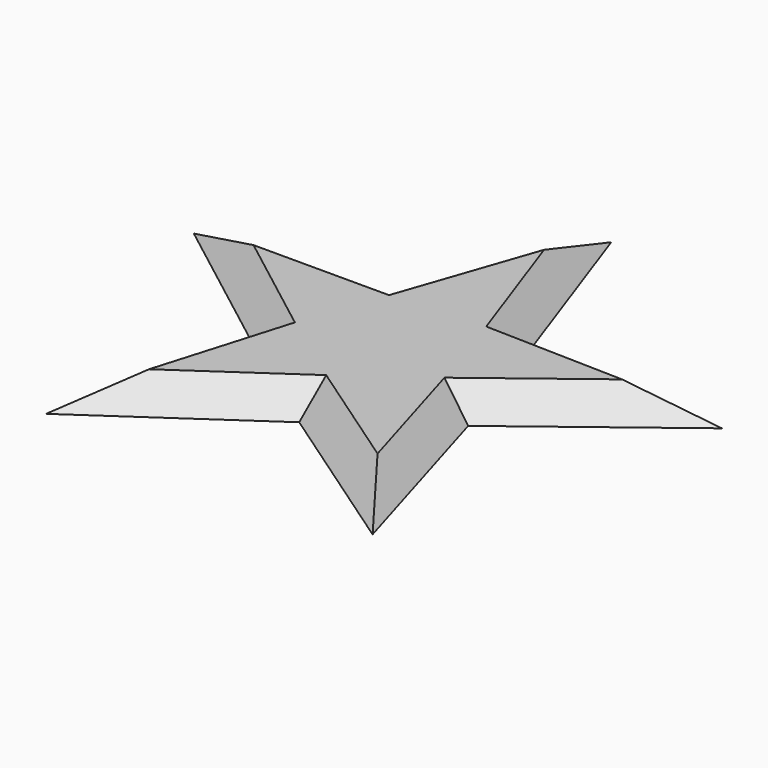
from build123d import *

# Parameters (mm, degrees)
F1_DEPTH      = 5
F2_T4_DEPTH   = 68.6680055615
F2_T9_DEPTH   = 69.5804590238
F2_T14_DEPTH  = 68.6556539851
F2_T19_DEPTH  = 68.6680055615
F2_T24_DEPTH  = 68.6680055615
F2_T29_DEPTH  = 68.6680055615
F2_T34_DEPTH  = 68.6680055615
F2_T39_DEPTH  = 68.6680055615
F2_T44_DEPTH  = 68.6680055615
F2_T49_DEPTH  = 68.6680055615
F2_T55_DEPTH  = 68.6680055615
F2_T59_DEPTH  = 68.6680055615
F2_T66_DEPTH  = 69.5804590238
F2_T70_DEPTH  = 68.6556539851
F2_T77_DEPTH  = 68.6680055615
F2_T81_DEPTH  = 68.6680055615
F2_T88_DEPTH  = 68.6680055615
F2_T92_DEPTH  = 68.6680055615
F2_T99_DEPTH  = 68.6680055615
F2_T103_DEPTH = 68.6680055615


# Not quite as in the source:
# - a fillet or chamfer that OpenCascade refuses, or shapes differently, is made with other operations: its cross-section is extruded or revolved along the edge and cut away or added


with BuildPart() as f1:
    # F0 (on Top) → F1 (new body)
    with BuildSketch(Plane.XY):
        Polygon((0, 0), (0, 52.987328628), (-12.5984860432, 16.3739850326), align=None)
        Polygon((12.5984860432, 17.3403284151), (0, 52.987328628), (0, 0), align=None)
        Polygon((0, 0), (-12.5984860432, 16.3739850326), (-50.3939441727, 16.3739850326), align=None)
        Polygon((50.3939441727, 16.3739850326), (12.5984860432, 17.3403284151), (0, 0), align=None)
        Polygon((20.3847786247, -6.6234160785), (0, 0), (31.1451703259, -42.8676493466), align=None)
        Polygon((0, -21.4338246733), (0, 0), (-31.1451703259, -42.8676493466), align=None)
        Polygon((-20.3847786247, -6.6234160785), (0, 0), (-50.3939441727, 16.3739850326), align=None)
        Polygon((50.3939441727, 16.3739850326), (0, 0), (20.3847786247, -6.6234160785), align=None)
        Polygon((31.1451703259, -42.8676493466), (0, 0), (0, -21.4338246733), align=None)
        Polygon((-31.1451703259, -42.8676493466), (0, 0), (-20.3847786247, -6.6234160785), align=None)
    extrude(amount=F1_DEPTH)

    # F2: chamfer of 6 on 10 edges, made by hand


with BuildPart() as f2_tool2:
    # F2_s3 → F2_t4 (new body)
    with BuildSketch(Plane(origin=(1.0926214012, -3.0915361725, 0), x_dir=(0, 0, 1), z_dir=(-0.3332244354, 0.9428475357, 0))):
        Polygon((-1, 17.6566726657), (5, 11.6566726657), (5, 17.6566726657), align=None)
    extrude(amount=F2_T4_DEPTH)

    split(bisect_by=Plane(origin=(0.451293236, 17.6509043406, 0), x_dir=(0, 0, 1), z_dir=(0.025559359, 0.9996733062, 0)), keep=Keep.TOP)


with BuildPart() as f1_1:
    add(f1.part)

    # F2_t1: cut F2_tool2
    add(f2_tool2.part, mode=Mode.SUBTRACT)


with BuildPart() as f2_tool7:
    # F2_s8 → F2_t9 (new body)
    with BuildSketch(Plane(origin=(21.3229816345, 61.9682119253, 0), x_dir=(0, 0, 1), z_dir=(-0.3253719116, -0.9455861247, 0))):
        Polygon((-1, 17.2405884042), (5, 11.2405884042), (5, 17.2405884042), align=None)
    extrude(amount=F2_T9_DEPTH)

    split(bisect_by=Plane.XZ.offset(-16.3739850326), keep=Keep.BOTTOM)


with BuildPart() as f1_2:
    add(f1_1.part)

    # F2_t6: cut F2_tool7
    add(f2_tool7.part, mode=Mode.SUBTRACT)


with BuildPart() as f2_tool12:
    # F2_s13 → F2_t14 (new body)
    with BuildSketch(Plane.YZ.offset(2.8316118846)):
        Polygon((16.3739850326, -1), (10.3739850326, 5), (16.3739850326, 5), align=None)
    extrude(amount=-F2_T14_DEPTH)

    split(bisect_by=Plane(origin=(-16.3024611761, 5.6096032055, 0), x_dir=(0, 0, 1), z_dir=(-0.9455861247, 0.3253719116, 0)), keep=Keep.TOP)


with BuildPart() as f1_3:
    add(f1_2.part)

    # F2_t11: cut F2_tool12
    add(f2_tool12.part, mode=Mode.SUBTRACT)


with BuildPart() as f2_tool17:
    # F2_s18 → F2_t19 (new body)
    with BuildSketch(Plane(origin=(-51.9012195214, 39.7742870116, 0), x_dir=(0, 0, 1), z_dir=(0.7937292793, -0.6082711823, 0))):
        Polygon((-1, 17.6566726657), (5, 11.6566726657), (5, 17.6566726657), align=None)
    extrude(amount=F2_T19_DEPTH)

    split(bisect_by=Plane(origin=(-16.926464871, 5.0252240345, 0), x_dir=(0, 0, 1), z_dir=(-0.9586440884, 0.2846076455, 0)), keep=Keep.TOP)


with BuildPart() as f1_4:
    add(f1_3.part)

    # F2_t16: cut F2_tool17
    add(f2_tool17.part, mode=Mode.SUBTRACT)


with BuildPart() as f2_tool22:
    # F2_s23 → F2_t24 (new body)
    with BuildSketch(Plane(origin=(0.9332100871, 3.1433320482, 0), x_dir=(0, 0, 1), z_dir=(-0.2846076455, -0.9586440884, 0))):
        Polygon((-1, 17.6566726657), (5, 11.6566726657), (5, 17.6566726657), align=None)
    extrude(amount=F2_T24_DEPTH)

    split(bisect_by=Plane(origin=(-10.7400451584, -14.014618069, 0), x_dir=(0, 0, 1), z_dir=(-0.6082711823, -0.7937292793, 0)), keep=Keep.TOP)


with BuildPart() as f1_5:
    add(f1_4.part)

    # F2_t21: cut F2_tool22
    add(f2_tool22.part, mode=Mode.SUBTRACT)


with BuildPart() as f2_tool27:
    # F2_s28 → F2_t29 (new body)
    with BuildSketch(Plane(origin=(-53.8659537043, -37.0700624038, 0), x_dir=(0, 0, 1), z_dir=(0.8237761079, 0.5669152707, 0))):
        Polygon((-1, 17.6566726657), (5, 11.6566726657), (5, 17.6566726657), align=None)
    extrude(amount=F2_T29_DEPTH)

    split(bisect_by=Plane(origin=(-10.0098373636, -14.5451450862, 0), x_dir=(0, 0, 1), z_dir=(-0.5669152707, -0.8237761079, 0)), keep=Keep.TOP)


with BuildPart() as f1_6:
    add(f1_5.part)

    # F2_t26: cut F2_tool27
    add(f2_tool27.part, mode=Mode.SUBTRACT)


with BuildPart() as f2_tool32:
    # F2_s33 → F2_t34 (new body)
    with BuildSketch(Plane(origin=(-2.7011086511, 1.8588785563, 0), x_dir=(0, 0, 1), z_dir=(0.8237761079, -0.5669152707, 0))):
        Polygon((-1, 17.6566726657), (5, 11.6566726657), (5, 17.6566726657), align=None)
    extrude(amount=F2_T34_DEPTH)

    split(bisect_by=Plane(origin=(10.0098373636, -14.5451450862, 0), x_dir=(0, 0, 1), z_dir=(0.5669152707, -0.8237761079, 0)), keep=Keep.TOP)


with BuildPart() as f1_7:
    add(f1_6.part)

    # F2_t31: cut F2_tool32
    add(f2_tool32.part, mode=Mode.SUBTRACT)


with BuildPart() as f2_tool37:
    # F2_s38 → F2_t39 (new body)
    with BuildSketch(Plane(origin=(18.6102292957, -62.6848455422, 0), x_dir=(0, 0, 1), z_dir=(-0.2846076455, 0.9586440884, 0))):
        Polygon((-1, 17.6566726657), (5, 11.6566726657), (5, 17.6566726657), align=None)
    extrude(amount=F2_T39_DEPTH)

    split(bisect_by=Plane(origin=(10.7400451584, -14.014618069, 0), x_dir=(0, 0, 1), z_dir=(0.6082711823, -0.7937292793, 0)), keep=Keep.TOP)


with BuildPart() as f1_8:
    add(f1_7.part)

    # F2_t36: cut F2_tool37
    add(f2_tool37.part, mode=Mode.SUBTRACT)


with BuildPart() as f2_tool42:
    # F2_s43 → F2_t44 (new body)
    with BuildSketch(Plane(origin=(-2.6025870408, -1.9944819195, 0), x_dir=(0, 0, 1), z_dir=(0.7937292793, 0.6082711823, 0))):
        Polygon((-1, 17.6566726657), (5, 11.6566726657), (5, 17.6566726657), align=None)
    extrude(amount=F2_T44_DEPTH)

    split(bisect_by=Plane(origin=(16.926464871, 5.0252240345, 0), x_dir=(0, 0, 1), z_dir=(0.9586440884, 0.2846076455, 0)), keep=Keep.TOP)


with BuildPart() as f1_9:
    add(f1_8.part)

    # F2_t41: cut F2_tool42
    add(f2_tool42.part, mode=Mode.SUBTRACT)


with BuildPart() as f2_tool47:
    # F2_s48 → F2_t49 (new body)
    with BuildSketch(Plane(origin=(65.3677079475, -1.6713027209, 0), x_dir=(0, 0, 1), z_dir=(-0.9996733062, 0.025559359, 0))):
        Polygon((-1, 17.6566726657), (5, 11.6566726657), (5, 17.6566726657), align=None)
    extrude(amount=F2_T49_DEPTH)

    split(bisect_by=Plane(origin=(16.6475503122, 5.8836347802, 0), x_dir=(0, 0, 1), z_dir=(0.9428475357, 0.3332244354, 0)), keep=Keep.TOP)


with BuildPart() as f1_10:
    add(f1_9.part)

    # F2_t46: cut F2_tool47
    add(f2_tool47.part, mode=Mode.SUBTRACT)


with BuildPart() as f2_tool53:
    # F2_s54 → F2_t55 (new body)
    with BuildSketch(Plane(origin=(1.0926214012, -3.0915361725, 0), x_dir=(0, 0, 1), z_dir=(-0.3332244354, 0.9428475357, 0))):
        Polygon((-1, 17.6566726657), (5, 11.6566726657), (5, 17.6566726657), align=None)
    extrude(amount=F2_T55_DEPTH)

    split(bisect_by=Plane(origin=(0.451293236, 17.6509043406, 0), x_dir=(0, 0, 1), z_dir=(-0.025559359, -0.9996733062, 0)), keep=Keep.TOP)


with BuildPart() as f2_tool57:
    # F2_s58 → F2_t59 (new body)
    with BuildSketch(Plane(origin=(65.3677079475, -1.6713027209, 0), x_dir=(0, 0, 1), z_dir=(-0.9996733062, 0.025559359, 0))):
        Polygon((-1, 17.6566726657), (5, 11.6566726657), (5, 17.6566726657), align=None)
    extrude(amount=F2_T59_DEPTH)

    split(bisect_by=Plane(origin=(16.6475503122, 5.8836347802, 0), x_dir=(0, 0, 1), z_dir=(-0.9428475357, -0.3332244354, 0)), keep=Keep.TOP)


with BuildPart() as f2_tool53_1:
    add(f2_tool53.part)

    # F2_t61: intersect F2_tool57
    add(f2_tool57.part, mode=Mode.INTERSECT)


with BuildPart() as f1_11:
    add(f1_10.part)

    # F2_t51: cut F2_tool53
    add(f2_tool53_1.part, mode=Mode.SUBTRACT)


with BuildPart() as f2_tool64:
    # F2_s65 → F2_t66 (new body)
    with BuildSketch(Plane(origin=(21.3229816345, 61.9682119253, 0), x_dir=(0, 0, 1), z_dir=(-0.3253719116, -0.9455861247, 0))):
        Polygon((-1, 17.2405884042), (5, 11.2405884042), (5, 17.2405884042), align=None)
    extrude(amount=F2_T66_DEPTH)

    split(bisect_by=Plane.XZ.offset(-16.3739850326), keep=Keep.TOP)


with BuildPart() as f2_tool68:
    # F2_s69 → F2_t70 (new body)
    with BuildSketch(Plane.YZ.offset(2.8316118846)):
        Polygon((16.3739850326, -1), (10.3739850326, 5), (16.3739850326, 5), align=None)
    extrude(amount=-F2_T70_DEPTH)

    split(bisect_by=Plane(origin=(-16.3024611761, 5.6096032055, 0), x_dir=(0, 0, 1), z_dir=(0.9455861247, -0.3253719116, 0)), keep=Keep.TOP)


with BuildPart() as f2_tool64_1:
    add(f2_tool64.part)

    # F2_t72: intersect F2_tool68
    add(f2_tool68.part, mode=Mode.INTERSECT)


with BuildPart() as f1_12:
    add(f1_11.part)

    # F2_t62: cut F2_tool64
    add(f2_tool64_1.part, mode=Mode.SUBTRACT)


with BuildPart() as f2_tool75:
    # F2_s76 → F2_t77 (new body)
    with BuildSketch(Plane(origin=(-51.9012195214, 39.7742870116, 0), x_dir=(0, 0, 1), z_dir=(0.7937292793, -0.6082711823, 0))):
        Polygon((-1, 17.6566726657), (5, 11.6566726657), (5, 17.6566726657), align=None)
    extrude(amount=F2_T77_DEPTH)

    split(bisect_by=Plane(origin=(-16.926464871, 5.0252240345, 0), x_dir=(0, 0, 1), z_dir=(0.9586440884, -0.2846076455, 0)), keep=Keep.TOP)


with BuildPart() as f2_tool79:
    # F2_s80 → F2_t81 (new body)
    with BuildSketch(Plane(origin=(0.9332100871, 3.1433320482, 0), x_dir=(0, 0, 1), z_dir=(-0.2846076455, -0.9586440884, 0))):
        Polygon((-1, 17.6566726657), (5, 11.6566726657), (5, 17.6566726657), align=None)
    extrude(amount=F2_T81_DEPTH)

    split(bisect_by=Plane(origin=(-10.7400451584, -14.014618069, 0), x_dir=(0, 0, 1), z_dir=(0.6082711823, 0.7937292793, 0)), keep=Keep.TOP)


with BuildPart() as f2_tool75_1:
    add(f2_tool75.part)

    # F2_t83: intersect F2_tool79
    add(f2_tool79.part, mode=Mode.INTERSECT)


with BuildPart() as f1_13:
    add(f1_12.part)

    # F2_t73: cut F2_tool75
    add(f2_tool75_1.part, mode=Mode.SUBTRACT)


with BuildPart() as f2_tool86:
    # F2_s87 → F2_t88 (new body)
    with BuildSketch(Plane(origin=(-53.8659537043, -37.0700624038, 0), x_dir=(0, 0, 1), z_dir=(0.8237761079, 0.5669152707, 0))):
        Polygon((-1, 17.6566726657), (5, 11.6566726657), (5, 17.6566726657), align=None)
    extrude(amount=F2_T88_DEPTH)

    split(bisect_by=Plane(origin=(-10.0098373636, -14.5451450862, 0), x_dir=(0, 0, 1), z_dir=(0.5669152707, 0.8237761079, 0)), keep=Keep.TOP)


with BuildPart() as f2_tool90:
    # F2_s91 → F2_t92 (new body)
    with BuildSketch(Plane(origin=(-2.7011086511, 1.8588785563, 0), x_dir=(0, 0, 1), z_dir=(0.8237761079, -0.5669152707, 0))):
        Polygon((-1, 17.6566726657), (5, 11.6566726657), (5, 17.6566726657), align=None)
    extrude(amount=F2_T92_DEPTH)

    split(bisect_by=Plane(origin=(10.0098373636, -14.5451450862, 0), x_dir=(0, 0, 1), z_dir=(-0.5669152707, 0.8237761079, 0)), keep=Keep.TOP)


with BuildPart() as f2_tool86_1:
    add(f2_tool86.part)

    # F2_t94: intersect F2_tool90
    add(f2_tool90.part, mode=Mode.INTERSECT)


with BuildPart() as f1_14:
    add(f1_13.part)

    # F2_t84: cut F2_tool86
    add(f2_tool86_1.part, mode=Mode.SUBTRACT)


with BuildPart() as f2_tool97:
    # F2_s98 → F2_t99 (new body)
    with BuildSketch(Plane(origin=(18.6102292957, -62.6848455422, 0), x_dir=(0, 0, 1), z_dir=(-0.2846076455, 0.9586440884, 0))):
        Polygon((-1, 17.6566726657), (5, 11.6566726657), (5, 17.6566726657), align=None)
    extrude(amount=F2_T99_DEPTH)

    split(bisect_by=Plane(origin=(10.7400451584, -14.014618069, 0), x_dir=(0, 0, 1), z_dir=(-0.6082711823, 0.7937292793, 0)), keep=Keep.TOP)


with BuildPart() as f2_tool101:
    # F2_s102 → F2_t103 (new body)
    with BuildSketch(Plane(origin=(-2.6025870408, -1.9944819195, 0), x_dir=(0, 0, 1), z_dir=(0.7937292793, 0.6082711823, 0))):
        Polygon((-1, 17.6566726657), (5, 11.6566726657), (5, 17.6566726657), align=None)
    extrude(amount=F2_T103_DEPTH)

    split(bisect_by=Plane(origin=(16.926464871, 5.0252240345, 0), x_dir=(0, 0, 1), z_dir=(-0.9586440884, -0.2846076455, 0)), keep=Keep.TOP)


with BuildPart() as f2_tool97_1:
    add(f2_tool97.part)

    # F2_t105: intersect F2_tool101
    add(f2_tool101.part, mode=Mode.INTERSECT)


with BuildPart() as f1_15:
    add(f1_14.part)

    # F2_t95: cut F2_tool97
    add(f2_tool97_1.part, mode=Mode.SUBTRACT)


solid = f1_15.part
